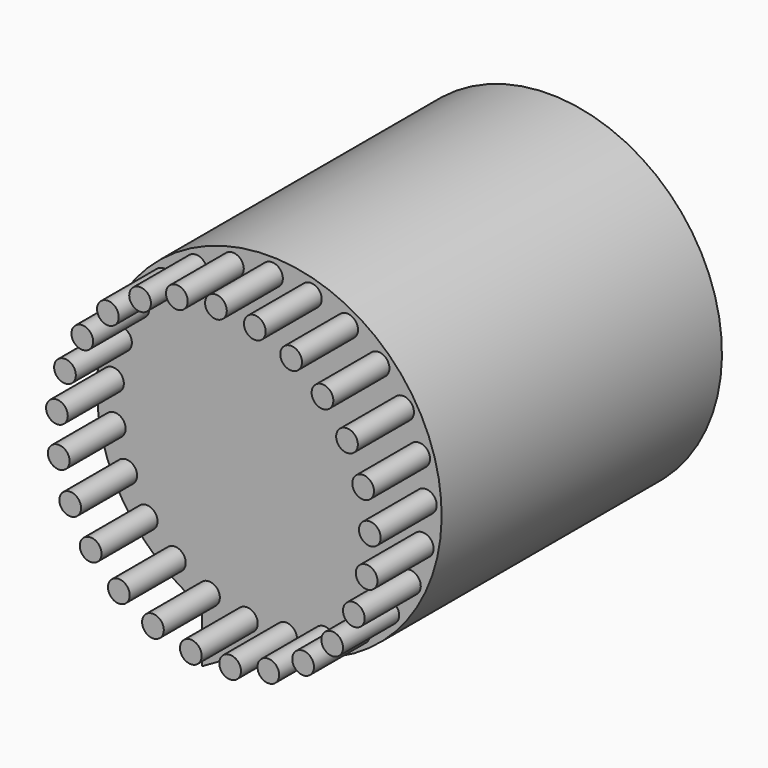
from build123d import *

# Parameters (mm, degrees)
F0_R            = 62.480427788
F1_DEPTH        = 63.5
F2_R            = 3.934558481
F3_DEPTH        = 25.4
F3_COPIES_COUNT = 25
F5_DEPTH        = 127


# Not quite as in the source:
# - a pattern or mirror of a feature is missing from the dataset's text; its kind, count and spacing are read off the source's solid


with BuildPart() as f1:
    # F0 (on Front) → F1 (new body, symmetric)
    with BuildSketch(Plane.XZ):
        Circle(F0_R)
    extrude(amount=F1_DEPTH, both=True)

    # F2 (on face) → F3 (join)
    with BuildSketch(Plane.XZ.offset(63.5)):
        with Locations((-38.1652005017, 42.0956611633)):
            Circle(F2_R)
    f3 = extrude(amount=F3_DEPTH)

    # F3_copies: F3 ×25 about axis
    f3_copies_axis = Axis((0, 0, 0), (0, 1, 0))
    for i in range(1, F3_COPIES_COUNT):
        add(f3.rotate(f3_copies_axis, i * 360 / F3_COPIES_COUNT))

    # F4 (on face) → F5 (join)
    with BuildSketch(Plane(origin=(0, 63.5, 0), x_dir=(-1, 0, 0), z_dir=(0, 1, 0))):
        Polygon((24.3383341717, -76.4241799678), (24.3383341717, -57.5451939463), (0, -62.480427788), align=None)
    extrude(amount=-F5_DEPTH)


solid = f1.part
